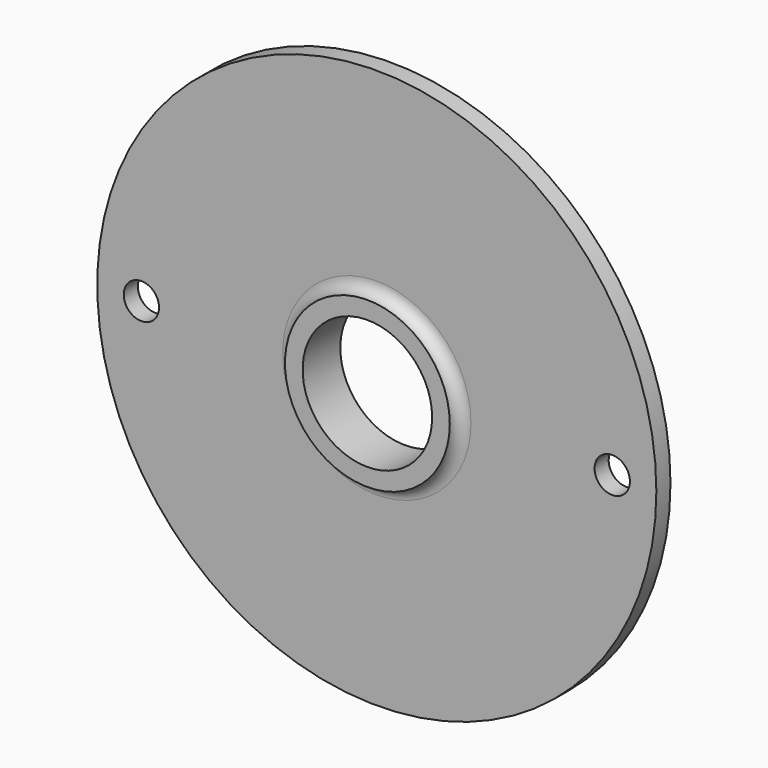
from build123d import *

# Parameters (mm, degrees)
F0_R     = 22.225
F0_R_2   = 17.4625
F1_DEPTH = 12.7
F2_START = 4.7625
F0_R_3   = 75.40625
F0_R_4   = 4.7625
F2_DEPTH = 4.7625
F3_R     = 3.17499


# Not quite as in the source:
# - a fillet or chamfer is up to 0.001 mm smaller than in the source, because OpenCascade refuses the exact size


with BuildPart() as f1:
    # F0 (on Front) → F1 (new body)
    with BuildSketch(Plane.XZ):
        Circle(F0_R)
        Circle(F0_R_2, mode=Mode.SUBTRACT)
    extrude(amount=F1_DEPTH)

    # F0 (on Front) → F2 (join)
    with BuildSketch(Plane.XZ.offset(F2_START)):
        Circle(F0_R_3)
        with Locations((-63.5, 0)):
            Circle(F0_R_4, mode=Mode.SUBTRACT)
        Circle(F0_R, mode=Mode.SUBTRACT)
        with Locations((63.5, 0)):
            Circle(F0_R_4, mode=Mode.SUBTRACT)
    extrude(amount=F2_DEPTH)

    # F3 (radius 3.175 in the source; OpenCascade refuses exactly that, so slightly less here)
    f3_edges = [f1.edges().sort_by_distance(p)[0] for p in [
        (-22.225, -9.525, 0),
        (-22.225, -4.7625, 0),
    ]]
    fillet(f3_edges, radius=F3_R)


solid = f1.part
